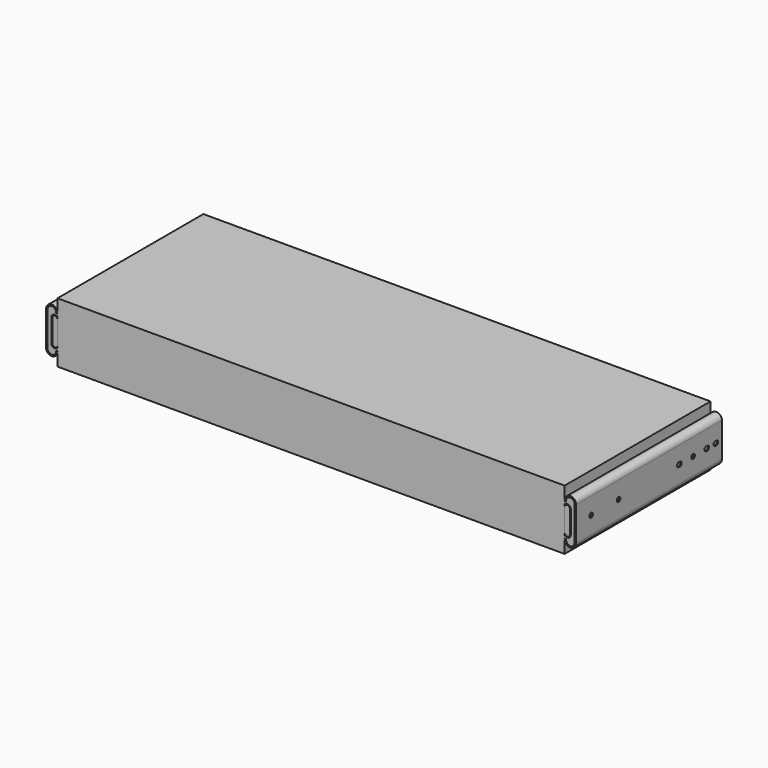
from build123d import *

# Parameters (mm, degrees)
F1_DEPTH       = 304.8
F2_R           = 2.5908
F2_R_2         = 4.7498
F3_DEPTH       = 25.4
F4_R           = 3.683
F5_DEPTH       = 25.4
F6_DEPTH       = 3.175
F7_DEPTH       = 3.175
F9_W           = 3.175
F9_H           = 3.175
F9_W_2         = 841.375
F9_H_2         = 94.234
F10_DEPTH      = 304.8
F11_R          = 2.5908
F11_R_2        = 4.7498
F12_DEPTH      = 22.226
F12_DEPTH_BACK = 863.601
F13_W          = 847.725
F13_H          = 100.584
F14_DEPTH      = 3.175


with BuildPart() as f1:
    # F0 (on Front) → F1 (new body)
    with BuildSketch(Plane.XZ):
        with BuildLine():
            Line((-442.9125, 66.675), (-442.9125, 9.525))
            ThreePointArc((-442.9125, 9.525), (-433.3875, 0), (-423.8625, 9.525))
            Line((-423.8625, 9.525), (-424.6924043996, 9.525))
            ThreePointArc((-424.6924043996, 9.525), (-425.2275505404, 9.3174732258), (-425.482867636, 8.8034090909))
            ThreePointArc((-425.482867636, 8.8034090909), (-433.7486695314, 1.5957211665), (-441.325, 9.525))
            Line((-441.325, 9.525), (-441.325, 66.675))
            ThreePointArc((-441.325, 66.675), (-433.7486695314, 74.6042788335), (-425.482867636, 67.3965909091))
            ThreePointArc((-425.482867636, 67.3965909091), (-425.2275505404, 66.8825267742), (-424.6924043996, 66.675))
            Line((-424.6924043996, 66.675), (-423.8625, 66.675))
            ThreePointArc((-423.8625, 66.675), (-433.3875, 76.2), (-442.9125, 66.675))
        make_face()
    extrude(amount=-F1_DEPTH)

    # F4 (on face) → F5 (cut)
    with BuildSketch(Plane(origin=(-442.9125, 0, 0), x_dir=(0, -1, 0), z_dir=(-1, 0, 0))):
        with Locations((-88.9, 38.1)):
            Circle(F4_R)
        with Locations((-31.75, 38.1)):
            Circle(F4_R)
        with Locations((-244.602, 38.1)):
            Circle(F4_R)
        with BuildLine():
            ThreePointArc((-293.243, 41.783), (-296.926, 38.1), (-293.243, 34.417))
            Line((-293.243, 34.417), (-290.957, 34.417))
            ThreePointArc((-290.957, 34.417), (-287.274, 38.1), (-290.957, 41.783))
            Line((-290.957, 41.783), (-293.243, 41.783))
        make_face()
        with BuildLine():
            ThreePointArc((-274.193, 41.783), (-277.876, 38.1), (-274.193, 34.417))
            Line((-274.193, 34.417), (-271.907, 34.417))
            ThreePointArc((-271.907, 34.417), (-268.224, 38.1), (-271.907, 41.783))
            Line((-271.907, 41.783), (-274.193, 41.783))
        make_face()
        with BuildLine():
            ThreePointArc((-217.043, 41.783), (-220.726, 38.1), (-217.043, 34.417))
            Line((-217.043, 34.417), (-214.757, 34.417))
            ThreePointArc((-214.757, 34.417), (-211.074, 38.1), (-214.757, 41.783))
            Line((-214.757, 41.783), (-217.043, 41.783))
        make_face()
    extrude(amount=-F5_DEPTH, mode=Mode.SUBTRACT)


with BuildPart() as f1b:
    # F0 (on Front) → F1, piece 2 (new body)
    with BuildSketch(Plane.XZ):
        with BuildLine():
            Line((-440.53125, 66.6749998859), (-440.53125, 9.5249998953))
            ThreePointArc((-440.53125, 9.5249998953), (-433.3874999476, 2.38125), (-426.24375, 9.525))
            ThreePointArc((-426.24375, 9.525), (-426.0112660076, 10.0862660076), (-425.45, 10.31875))
            Line((-425.45, 10.31875), (-423.8625, 10.31875))
            Line((-423.8625, 10.31875), (-423.8625, 15.1812246945))
            ThreePointArc((-423.8625, 15.1812246945), (-430.4018989001, 13.6865136661), (-434.18125, 19.2285714334))
            Line((-434.18125, 19.2285714334), (-434.18125, 56.9714283477))
            ThreePointArc((-434.18125, 56.9714283477), (-430.4018989001, 62.5134861151), (-423.8625, 61.0187750867))
            Line((-423.8625, 61.0187750867), (-423.8625, 65.88125))
            Line((-423.8625, 65.88125), (-425.45, 65.88125))
            ThreePointArc((-425.45, 65.88125), (-426.0112660076, 66.1137339924), (-426.24375, 66.675))
            ThreePointArc((-426.24375, 66.675), (-433.387500057, 73.81875), (-440.53125, 66.6749998859))
        make_face()
    extrude(amount=-F1_DEPTH)


with BuildPart() as f1c:
    # F0 (on Front) → F1, piece 3 (new body)
    with BuildSketch(Plane.XZ):
        with BuildLine():
            Line((-432.59375, 56.9714283477), (-432.59375, 19.2285714334))
            ThreePointArc((-432.59375, 19.2285714334), (-428.228125, 14.8629464334), (-423.8625, 19.2285714334))
            Line((-423.8625, 19.2285714334), (-423.8625, 56.9714283477))
            ThreePointArc((-423.8625, 56.9714283477), (-428.228125, 61.3370533477), (-432.59375, 56.9714283477))
        make_face()
    extrude(amount=-F1_DEPTH)

    # F2 (on face) → F3 (cut)
    with BuildSketch(Plane.YZ.offset(-423.8625)):
        with BuildLine():
            ThreePointArc((48.2092, 35.0900998906), (50.8, 32.4992998906), (53.3908, 35.0900998906))
            Line((53.3908, 35.0900998906), (53.3908, 41.1098998906))
            ThreePointArc((53.3908, 41.1098998906), (50.8, 43.7006998906), (48.2092, 41.1098998906))
            Line((48.2092, 41.1098998906), (48.2092, 35.0900998906))
        make_face()
        with BuildLine():
            ThreePointArc((188.3156, 35.5091998906), (190.9064, 38.0999998906), (188.3156, 40.6907998906))
            Line((188.3156, 40.6907998906), (184.0484, 40.6907998906))
            ThreePointArc((184.0484, 40.6907998906), (181.4576, 38.0999998906), (184.0484, 35.5091998906))
            Line((184.0484, 35.5091998906), (188.3156, 35.5091998906))
        make_face()
        with BuildLine():
            ThreePointArc((208.9404, 40.6907998906), (206.3496, 38.0999998906), (208.9404, 35.5091998906))
            Line((208.9404, 35.5091998906), (213.2076, 35.5091998906))
            ThreePointArc((213.2076, 35.5091998906), (215.7984, 38.0999998906), (213.2076, 40.6907998906))
            Line((213.2076, 40.6907998906), (208.9404, 40.6907998906))
        make_face()
        with BuildLine():
            ThreePointArc((227.9904, 40.6907998906), (225.3996, 38.0999998906), (227.9904, 35.5091998906))
            Line((227.9904, 35.5091998906), (232.2576, 35.5091998906))
            ThreePointArc((232.2576, 35.5091998906), (234.8484, 38.0999998906), (232.2576, 40.6907998906))
            Line((232.2576, 40.6907998906), (227.9904, 40.6907998906))
        make_face()
        with BuildLine():
            ThreePointArc((251.3076, 35.5091998906), (253.8984, 38.0999998906), (251.3076, 40.6907998906))
            Line((251.3076, 40.6907998906), (247.0404, 40.6907998906))
            ThreePointArc((247.0404, 40.6907998906), (244.4496, 38.0999998906), (247.0404, 35.5091998906))
            Line((247.0404, 35.5091998906), (251.3076, 35.5091998906))
        make_face()
        with Locations((31.75, 38.0999998906)):
            Circle(F2_R)
        with Locations((69.85, 38.0999998906)):
            Circle(F2_R)
        with Locations((95.25, 38.0999998906)):
            Circle(F2_R)
        with Locations((12.7, 38.0999998906)):
            Circle(F2_R_2)
    extrude(amount=-F3_DEPTH, mode=Mode.SUBTRACT)

    # F6 (cut): a face of the model
    f6_faces = [f1c.faces().sort_by_distance(p)[0] for p in [
        (-428.228125, 0, 38.0999998906),
    ]]
    extrude(f6_faces, amount=-F6_DEPTH, mode=Mode.SUBTRACT)


with BuildPart() as f7:
    # F7 (new): a face of the model
    f7_faces = [f1c.part.faces().sort_by_distance(p)[0] for p in [
        (-428.228125, 3.175, 38.0999998906),
    ]]
    extrude(f7_faces, amount=F7_DEPTH)


with BuildPart() as f8_1:
    # F8: instance of F1c
    add(f1c.part.mirror(Plane.YZ))


with BuildPart() as f8_2:
    # F8: instance of F1b
    add(f1b.part.mirror(Plane.YZ))


with BuildPart() as f8_3:
    # F8: instance of F1
    add(f1.part.mirror(Plane.YZ))


with BuildPart() as f8_4:
    # F8: instance of F7
    add(f7.part.mirror(Plane.YZ))


with BuildPart() as f10:
    # F9 (on Front) → F10 (new body)
    with BuildSketch(Plane.XZ):
        with Locations((-422.275, 86.8044998906)):
            Rectangle(F9_W, F9_H)
        with Locations((0, 86.8044998906)):
            Rectangle(F9_W_2, F9_H)
        Polygon((-420.6875, 85.2169998906), (-423.8625, 85.2169998906), (-423.8625, 56.9714283477), (-423.8625, 19.2285714334), (-423.8625, -9.0170001094), (-420.6875, -9.0170001094), align=None)
        with Locations((422.275, 86.8044998906)):
            Rectangle(F9_W, F9_H)
        with Locations((-422.275, -10.6045001094)):
            Rectangle(F9_W, F9_H)
        with Locations((422.275, 38.0999998906)):
            Rectangle(F9_W, F9_H_2)
        with Locations((422.275, -10.6045001094)):
            Rectangle(F9_W, F9_H)
    extrude(amount=-F10_DEPTH)

    # F11 (on face) → F12 (cut, two sides)
    with BuildSketch(Plane.YZ.offset(-420.6875)) as f12_sk:
        with BuildLine():
            ThreePointArc((48.2092, 35.0900998906), (50.8, 32.4992998906), (53.3908, 35.0900998906))
            Line((53.3908, 35.0900998906), (53.3908, 41.1098998906))
            ThreePointArc((53.3908, 41.1098998906), (50.8, 43.7006998906), (48.2092, 41.1098998906))
            Line((48.2092, 41.1098998906), (48.2092, 35.0900998906))
        make_face()
        with BuildLine():
            ThreePointArc((188.3156, 35.5091998906), (190.9064, 38.0999998906), (188.3156, 40.6907998906))
            Line((188.3156, 40.6907998906), (184.0484, 40.6907998906))
            ThreePointArc((184.0484, 40.6907998906), (181.4576, 38.0999998906), (184.0484, 35.5091998906))
            Line((184.0484, 35.5091998906), (188.3156, 35.5091998906))
        make_face()
        with BuildLine():
            ThreePointArc((208.9404, 40.6907998906), (206.3496, 38.0999998906), (208.9404, 35.5091998906))
            Line((208.9404, 35.5091998906), (213.2076, 35.5091998906))
            ThreePointArc((213.2076, 35.5091998906), (215.7984, 38.0999998906), (213.2076, 40.6907998906))
            Line((213.2076, 40.6907998906), (208.9404, 40.6907998906))
        make_face()
        with BuildLine():
            ThreePointArc((227.9904, 40.6907998906), (225.3996, 38.0999998906), (227.9904, 35.5091998906))
            Line((227.9904, 35.5091998906), (232.2576, 35.5091998906))
            ThreePointArc((232.2576, 35.5091998906), (234.8484, 38.0999998906), (232.2576, 40.6907998906))
            Line((232.2576, 40.6907998906), (227.9904, 40.6907998906))
        make_face()
        with BuildLine():
            ThreePointArc((251.3076, 35.5091998906), (253.8984, 38.0999998906), (251.3076, 40.6907998906))
            Line((251.3076, 40.6907998906), (247.0404, 40.6907998906))
            ThreePointArc((247.0404, 40.6907998906), (244.4496, 38.0999998906), (247.0404, 35.5091998906))
            Line((247.0404, 35.5091998906), (251.3076, 35.5091998906))
        make_face()
        with Locations((31.75, 38.0999998906)):
            Circle(F11_R)
        with Locations((69.85, 38.0999998906)):
            Circle(F11_R)
        with Locations((95.25, 38.0999998906)):
            Circle(F11_R)
        with Locations((12.7, 38.0999998906)):
            Circle(F11_R_2)
    extrude(amount=-F12_DEPTH, mode=Mode.SUBTRACT)
    extrude(f12_sk.sketch, amount=F12_DEPTH_BACK, mode=Mode.SUBTRACT)

    # F13 (on face) → F14 (join)
    with BuildSketch(Plane.XZ):
        with Locations((0, 38.0999998906)):
            Rectangle(F13_W, F13_H)
    extrude(amount=-F14_DEPTH)


solid = Compound([f1.part, f1b.part, f1c.part, f7.part, f8_1.part, f8_2.part, f8_3.part, f8_4.part, f10.part])
